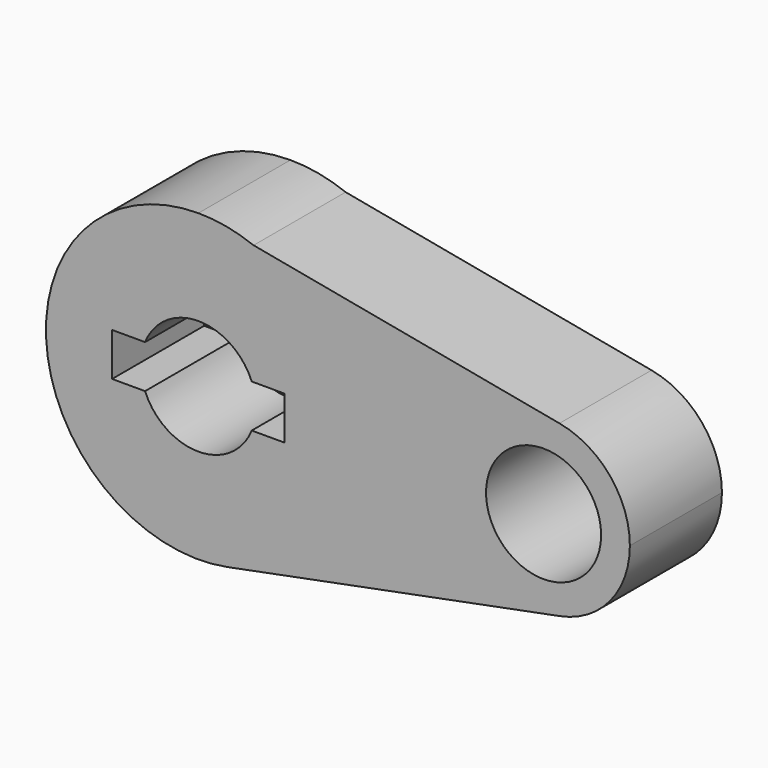
from build123d import *

# Parameters (mm, degrees)
F1_DEPTH = 25.4
F0_R     = 12.7
F2_DEPTH = 25.4


# Not quite as in the source:
# - the program builds the solid bodies; features that only make, move or delete a surface that nothing else refers to are left out


with BuildPart() as f1:
    # F0 (on Front) → F1 (new body)
    with BuildSketch(Plane.XZ):
        with BuildLine():
            Line((12.1809959468, 31.3732746576), (0, 33.655))
            ThreePointArc((0, 33.655), (-33.498646558, -3.2403246414), (6.4505416667, -33.0310389968))
            ThreePointArc((6.4505416667, -33.0310389968), (25.9783756689, -21.3958646146), (33.655, 0))
            ThreePointArc((33.655, 0), (27.7723823572, 19.0093083305), (12.1809959468, 31.3732746576))
        make_face()
        with BuildLine():
            ThreePointArc((-11.7732150983, 4.7625), (0, 12.7), (11.7732150983, 4.7625))
            Line((11.7732150983, 4.7625), (19.05, 4.7625))
            Line((19.05, 4.7625), (19.05, -4.7625))
            Line((19.05, -4.7625), (11.7732150983, -4.7625))
            ThreePointArc((11.7732150983, -4.7625), (0, -12.7), (-11.7732150983, -4.7625))
            Line((-11.7732150983, -4.7625), (-19.05, -4.7625))
            Line((-19.05, -4.7625), (-19.05, 4.7625))
            Line((-19.05, 4.7625), (-11.7732150983, 4.7625))
        make_face(mode=Mode.SUBTRACT)
    extrude(amount=F1_DEPTH)

    # F0 (on Front) → F2 (join)
    with BuildSketch(Plane.XZ):
        with BuildLine():
            Line((12.1809959468, 31.3732746576), (0, 33.655))
            ThreePointArc((0, 33.655), (-33.498646558, -3.2403246414), (6.4505416667, -33.0310389968))
            ThreePointArc((6.4505416667, -33.0310389968), (25.9783756689, -21.3958646146), (33.655, 0))
            ThreePointArc((33.655, 0), (27.7723823572, 19.0093083305), (12.1809959468, 31.3732746576))
        make_face()
        with BuildLine():
            ThreePointArc((-11.7732150983, 4.7625), (0, 12.7), (11.7732150983, 4.7625))
            Line((11.7732150983, 4.7625), (19.05, 4.7625))
            Line((19.05, 4.7625), (19.05, -4.7625))
            Line((19.05, -4.7625), (11.7732150983, -4.7625))
            ThreePointArc((11.7732150983, -4.7625), (0, -12.7), (-11.7732150983, -4.7625))
            Line((-11.7732150983, -4.7625), (-19.05, -4.7625))
            Line((-19.05, -4.7625), (-19.05, 4.7625))
            Line((-19.05, 4.7625), (-11.7732150983, 4.7625))
        make_face(mode=Mode.SUBTRACT)
        with BuildLine():
            ThreePointArc((12.1809959468, 31.3732746576), (6.1964290683, 33.0796507207), (0, 33.655))
            Line((0, 33.655), (12.1809959468, 31.3732746576))
        make_face()
        with BuildLine():
            ThreePointArc((33.655, 0), (25.9783756689, -21.3958646146), (6.4505416667, -33.0310389968))
            Line((6.4505416667, -33.0310389968), (79.85125, -18.6968145265))
            ThreePointArc((79.85125, -18.6968145265), (57.1501407243, -0.0732227913), (79.7074126802, 18.7243305966))
            Line((79.7074126802, 18.7243305966), (12.1809959468, 31.3732746576))
            ThreePointArc((12.1809959468, 31.3732746576), (27.7723823572, 19.0093083305), (33.655, 0))
        make_face()
        with BuildLine():
            ThreePointArc((79.7074126802, 18.7243305966), (57.1501407243, -0.0732227913), (79.85125, -18.6968145265))
            ThreePointArc((79.85125, -18.6968145265), (90.9047409447, -12.110866763), (95.25, 0))
            ThreePointArc((95.25, 0), (90.8580815859, 12.167298148), (79.7074126802, 18.7243305966))
        make_face()
        with Locations((76.2, 0)):
            Circle(F0_R, mode=Mode.SUBTRACT)
    extrude(amount=F2_DEPTH)


solid = f1.part
